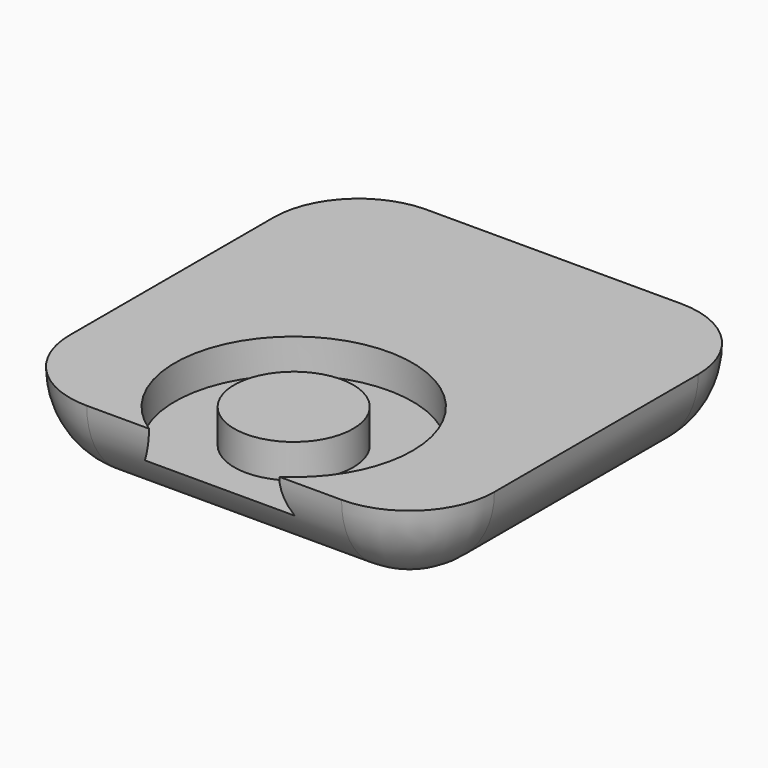
from build123d import *

# Parameters (mm, degrees)
F0_W     = 25
F0_H     = 25
F1_DEPTH = 5
F2_R     = 5
F3_R     = 4.99999
F5_START = 3
F4_R     = 3.5
F5_DEPTH = 22


# Not quite as in the source:
# - a fillet or chamfer is up to 0.001 mm smaller than in the source, because OpenCascade refuses the exact size


with BuildPart() as f1:
    # F0 (on Top) → F1 (new body)
    with BuildSketch(Plane.XY):
        with Locations((12.5, 0.6441110272)):
            Rectangle(F0_W, F0_H)
    extrude(amount=F1_DEPTH)

    # F2
    f2_edges = [f1.edges().sort_by_distance(p)[0] for p in [
        (0, 13.144111, 2.5),
        (25, 13.144111, 2.5),
        (0, -11.855889, 2.5),
        (25, -11.855889, 2.5),
    ]]
    fillet(f2_edges, radius=F2_R)

    # F3 (radius 5 in the source; OpenCascade refuses exactly that, so slightly less here)
    f3_edges = [f1.edges().sort_by_distance(p)[0] for p in [
        (12.5, -11.855889, 0),
        (0, 0.644111, 0),
        (25, 0.644111, 0),
        (12.5, 13.144111, 0),
    ]]
    fillet(f3_edges, radius=F3_R)

    # F4 (on Top) → F5 (cut)
    with BuildSketch(Plane.XY.offset(F5_START)):
        with BuildLine():
            ThreePointArc((19.5, -6), (9.1718039657, 0.1581743364), (8.6648253836, -11.8558889728))
            Line((8.6648253836, -11.8558889728), (16.3351746164, -11.8558889728))
            ThreePointArc((16.3351746164, -11.8558889728), (18.6581743364, -9.3281960343), (19.5, -6))
        make_face()
        with Locations((12.5, -6)):
            Circle(F4_R, mode=Mode.SUBTRACT)
    extrude(amount=F5_DEPTH, mode=Mode.SUBTRACT)


solid = f1.part
